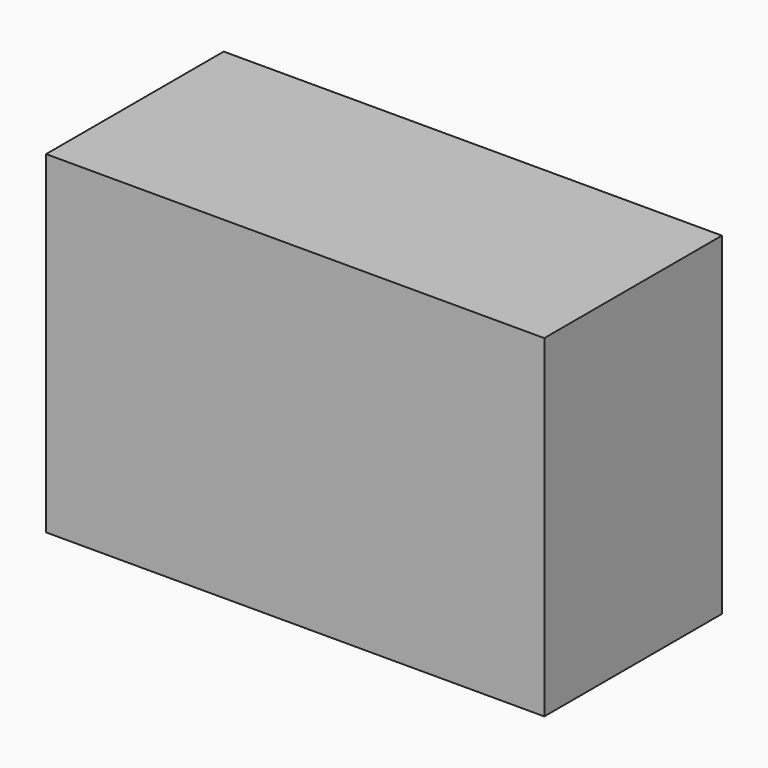
from build123d import *

# Parameters (mm, degrees)
F0_W     = 113.9825060964
F0_H     = 76.2000009418
F1_DEPTH = 50.8


# Not quite as in the source:
# - the program builds the solid bodies; features that only make, move or delete a surface that nothing else refers to are left out


with BuildPart() as f1:
    # F0 (on Front) → F1 (new body)
    with BuildSketch(Plane.XZ):
        Rectangle(F0_W, F0_H)
    extrude(amount=-F1_DEPTH)


solid = f1.part
